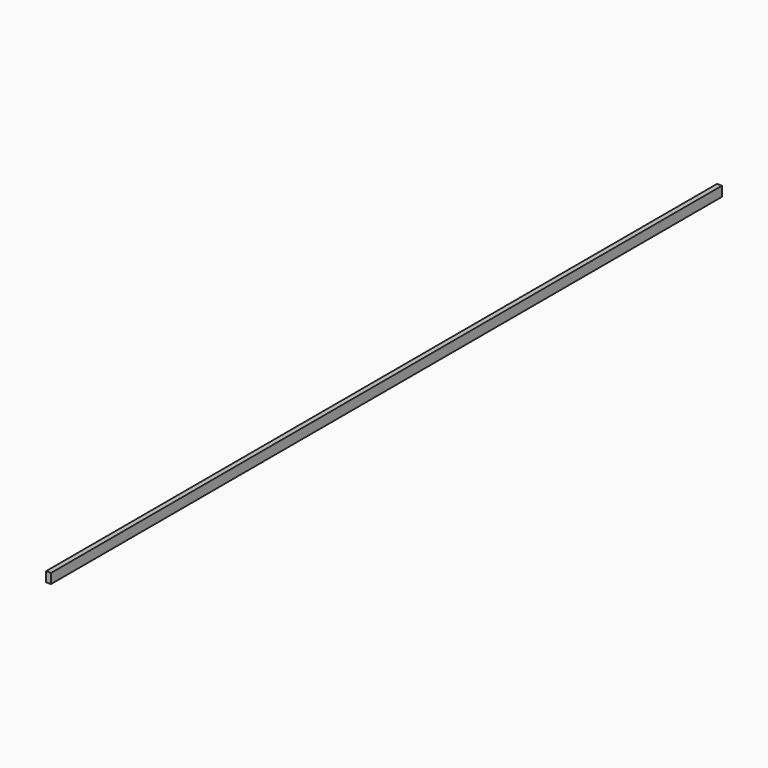
from build123d import *

# Parameters (mm, degrees)
F0_W     = 15.875
F0_H     = 31.75
F1_DEPTH = 25.4
F2_DEPTH = 2686.05


# Not quite as in the source:
# - a feature names something its author has since deleted; it is built from what else it names


with BuildPart() as f1:
    # F0 (on Front) → F1 (new body)
    with BuildSketch(Plane.XZ):
        with Locations((7.9375, -15.875)):
            Rectangle(F0_W, F0_H)
    extrude(amount=F1_DEPTH)

    # F2 (add): a face of the model
    f2_faces = [f1.faces().sort_by_distance(p)[0] for p in [
        (7.9375, 0, -15.875),
    ]]
    extrude(f2_faces, amount=F2_DEPTH)


solid = f1.part
